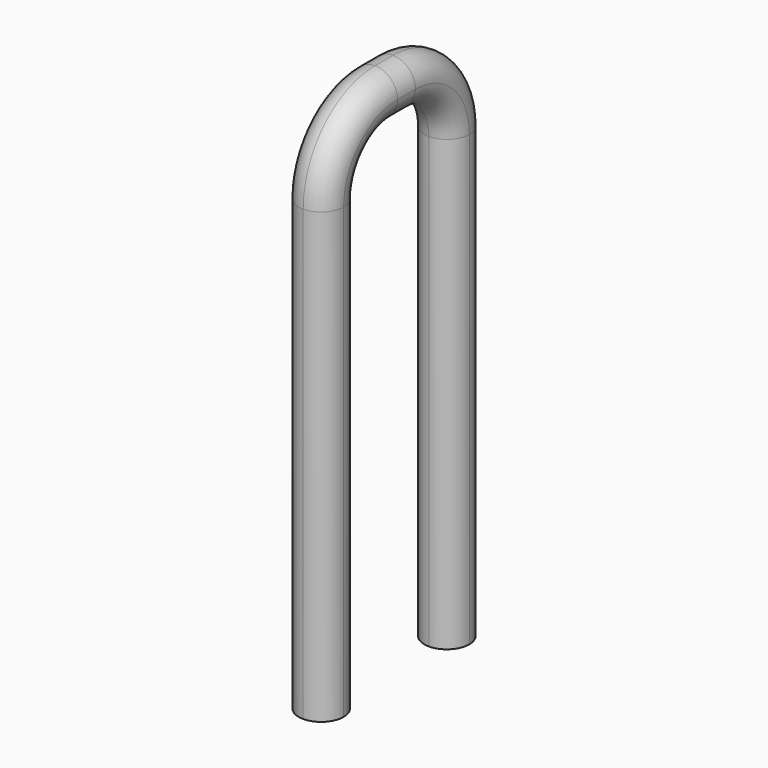
from build123d import *

# Parameters (mm, degrees)
F1_DEPTH = 101.6
F2_R     = 101.6
F3_R     = 203.2
F4_R     = 50.79999


# Not quite as in the source:
# - a fillet or chamfer is up to 0.001 mm smaller than in the source, because OpenCascade refuses the exact size


with BuildPart() as f1:
    # F0 (on Right) → F1 (new body)
    with BuildSketch(Plane.YZ):
        Polygon((-309.582978487, 0), (-207.982978487, 0), (-207.982978487, 1111.25), (-207.982978487, 1117.6), (-201.632978487, 1117.6), (46.017021513, 1117.6), (46.017021513, 0), (147.617021513, 0), (147.617021513, 1219.2), (-309.582978487, 1219.2), align=None)
    extrude(amount=F1_DEPTH)

    # F2
    f2_edges = [f1.edges().sort_by_distance(p)[0] for p in [
        (50.8, -207.982978, 1117.6),
        (50.8, 46.017022, 1117.6),
    ]]
    fillet(f2_edges, radius=F2_R)

    # F3
    f3_edges = [f1.edges().sort_by_distance(p)[0] for p in [
        (50.8, -309.582978, 1219.2),
        (50.8, 147.617022, 1219.2),
    ]]
    fillet(f3_edges, radius=F3_R)

    # F4 (radius 50.8 in the source; OpenCascade refuses exactly that, so slightly less here)
    f4_edges = [f1.edges().sort_by_distance(p)[0] for p in [
        (101.6, -207.982978, 508),
        (101.6, -309.582978, 508),
        (0, -309.582978, 508),
        (0, -207.982978, 508),
    ]]
    fillet(f4_edges, radius=F4_R)


solid = f1.part
